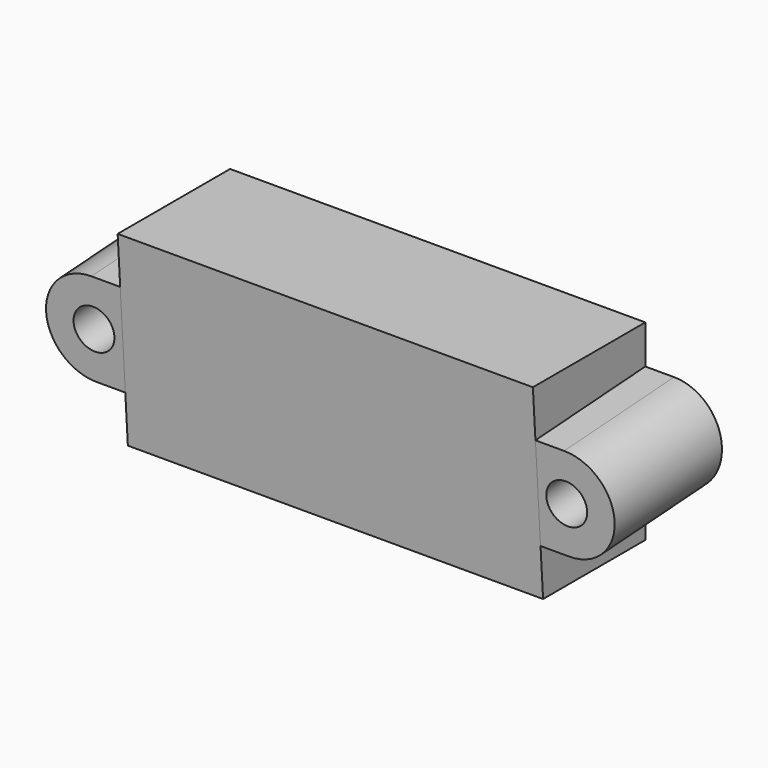
from build123d import *

# Parameters (mm, degrees)
F1_DEPTH = 16.25
F2_R     = 1.6
F3_REACH = 20.5813230926


with BuildPart() as f1:
    # F0 (on Right) → F1 (new body, symmetric)
    with BuildSketch(Plane.YZ):
        Polygon((-10, 0), (0, 0), (0, 15), (-11, 15), align=None)
    extrude(amount=F1_DEPTH, both=True)

    f3_end = Plane(origin=(0, 0, 7.5), x_dir=(0, 0, 1), z_dir=(0, 1, 0))
    # F2 (on face) → F3 (join, up to a plane its end follows)
    with BuildSketch(Plane(origin=(0, -9.9557522124, -0.6637168142), x_dir=(1, 0, 0), z_dir=(0, -0.9977851579, -0.0665190105))):
        with BuildLine():
            Line((-18.5, 4.4318382944), (-16.25, 4.4318382944))
            Line((-16.25, 4.4318382944), (-16.25, 11.9318382944))
            Line((-16.25, 11.9318382944), (-18.5, 11.9318382944))
            ThreePointArc((-18.5, 11.9318382944), (-22.25, 8.1818382944), (-18.5, 4.4318382944))
        make_face()
        with Locations((-18.5, 8.1818382944)):
            Circle(F2_R, mode=Mode.SUBTRACT)
        with BuildLine():
            Line((16.25, 4.4318382944), (18.5, 4.4318382944))
            ThreePointArc((18.5, 4.4318382944), (22.25, 8.1818382944), (18.5, 11.9318382944))
            Line((18.5, 11.9318382944), (16.25, 11.9318382944))
            Line((16.25, 11.9318382944), (16.25, 4.4318382944))
        make_face()
        with Locations((18.5, 8.1818382944)):
            Circle(F2_R, mode=Mode.SUBTRACT)
    f3_long = extrude(amount=-F3_REACH, mode=Mode.PRIVATE)
    add(split(f3_long, bisect_by=f3_end, keep=Keep.BOTTOM, mode=Mode.PRIVATE))


solid = f1.part
